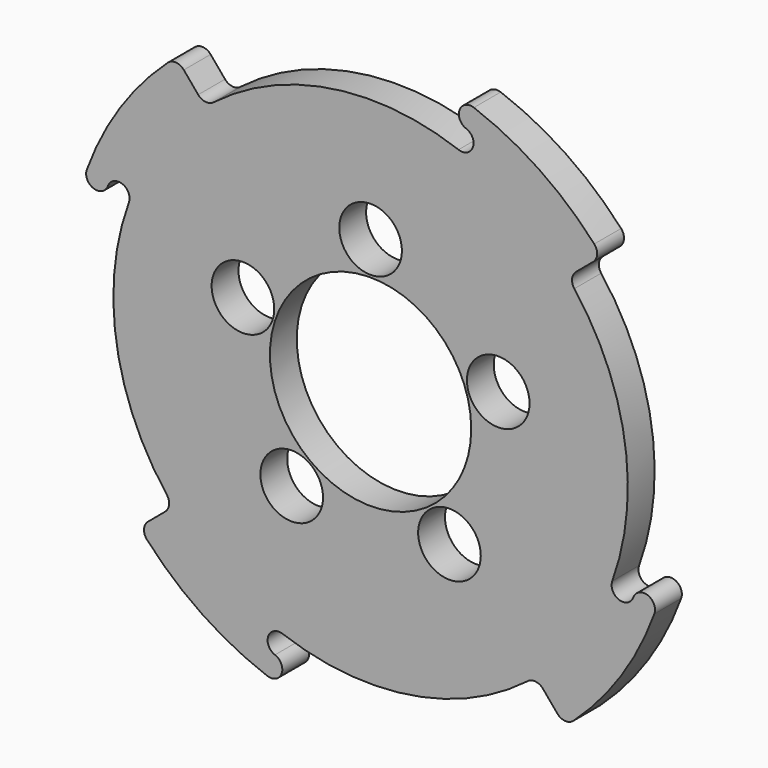
from build123d import *

# Parameters (mm, degrees)
F0_R     = 14
F0_R_2   = 45
F1_DEPTH = 15
F3_COUNT = 4
F4_R     = 14
F5_DEPTH = 15.001


# Not quite as in the source:
# - a feature names something its author has since deleted; it is built from what else it names


with BuildPart() as f1:
    # F0 (on Front) → F1 (new body)
    with BuildSketch(Plane.XZ):
        with BuildLine():
            ThreePointArc((-117.4615775982, 42.7525179157), (-111.0530137777, 45.740880303), (-108.0646513904, 39.3323164825))
            ThreePointArc((-108.0646513904, 39.3323164825), (-113.6444232454, -17.6052567496), (-91.0986302517, -70.1857504502))
            ThreePointArc((-91.0986302517, -70.1857504502), (-90.0886289945, -73.7767817278), (-91.8455022142, -77.0675270332))
            Line((-91.8455022142, -77.0675270332), (-99.5120922253, -83.500559884))
            ThreePointArc((-99.5120922253, -83.500559884), (-101.2865881138, -86.990889679), (-100.0019293376, -90.6896583342))
            ThreePointArc((-100.0019293376, -90.6896583342), (-75.2914558589, -112.0544362114), (-46.172719349, -126.8585038061))
            ThreePointArc((-46.172719349, -126.8585038061), (-39.7641555284, -123.8701414188), (-42.7525179157, -117.4615775982))
            ThreePointArc((-42.7525179157, -117.4615775982), (-45.740880303, -111.0530137777), (-39.3323164825, -108.0646513904))
            ThreePointArc((-39.3323164825, -108.0646513904), (17.6052567496, -113.6444232454), (70.1857504502, -91.0986302517))
            ThreePointArc((70.1857504502, -91.0986302517), (73.7767817278, -90.0886289945), (77.0675270332, -91.8455022142))
            Line((77.0675270332, -91.8455022142), (83.500559884, -99.5120922253))
            ThreePointArc((83.500559884, -99.5120922253), (86.990889679, -101.2865881138), (90.6896583342, -100.0019293376))
            ThreePointArc((90.6896583342, -100.0019293376), (112.0544362114, -75.2914558589), (126.8585038061, -46.172719349))
            ThreePointArc((126.8585038061, -46.172719349), (123.8701414188, -39.7641555284), (117.4615775982, -42.7525179157))
            ThreePointArc((117.4615775982, -42.7525179157), (111.0530137777, -45.740880303), (108.0646513904, -39.3323164825))
            ThreePointArc((108.0646513904, -39.3323164825), (113.6444232454, 17.6052567496), (91.0986302517, 70.1857504502))
            ThreePointArc((91.0986302517, 70.1857504502), (90.0886289945, 73.7767817278), (91.8455022142, 77.0675270332))
            Line((91.8455022142, 77.0675270332), (99.5120922253, 83.500559884))
            ThreePointArc((99.5120922253, 83.500559884), (101.2865881138, 86.990889679), (100.0019293376, 90.6896583342))
            ThreePointArc((100.0019293376, 90.6896583342), (75.2914558589, 112.0544362114), (46.172719349, 126.8585038061))
            ThreePointArc((46.172719349, 126.8585038061), (39.7641555284, 123.8701414188), (42.7525179157, 117.4615775982))
            ThreePointArc((42.7525179157, 117.4615775982), (45.740880303, 111.0530137777), (39.3323164825, 108.0646513904))
            ThreePointArc((39.3323164825, 108.0646513904), (-17.6052567496, 113.6444232454), (-70.1857504502, 91.0986302517))
            ThreePointArc((-70.1857504502, 91.0986302517), (-73.7767817278, 90.0886289945), (-77.0675270332, 91.8455022142))
            Line((-77.0675270332, 91.8455022142), (-83.500559884, 99.5120922253))
            ThreePointArc((-83.500559884, 99.5120922253), (-86.990889679, 101.2865881138), (-90.6896583342, 100.0019293376))
            ThreePointArc((-90.6896583342, 100.0019293376), (-112.0544362114, 75.2914558589), (-126.8585038061, 46.172719349))
            ThreePointArc((-126.8585038061, 46.172719349), (-123.8701414188, 39.7641555284), (-117.4615775982, 42.7525179157))
        make_face()
        with Locations((-35.2671151375, -48.5410196625)):
            Circle(F0_R, mode=Mode.SUBTRACT)
        with Locations((35.2671151375, -48.5410196625)):
            Circle(F0_R, mode=Mode.SUBTRACT)
        with Locations((-57.0633909777, 18.5410196625)):
            Circle(F0_R, mode=Mode.SUBTRACT)
        Circle(F0_R_2, mode=Mode.SUBTRACT)
        with Locations((57.0633909777, 18.5410196625)):
            Circle(F0_R, mode=Mode.SUBTRACT)
        with Locations((0, 60)):
            Circle(F0_R, mode=Mode.SUBTRACT)
    extrude(amount=F1_DEPTH)

    # F3: F1 ×4 about axis
    f3_axis = Axis((0, -15, 0), (0, -1, 0))


with BuildPart() as f1_1:
    add(f1.part)
    for i in range(1, F3_COUNT):
        add(f1.part.rotate(f3_axis, i * 360 / F3_COUNT))

    # F4 (on face) → F5 (cut, through all)
    with BuildSketch(Plane.XZ.offset(15)):
        with Locations((0, 60)):
            Circle(F4_R)
        with Locations((-57.0633909777, 18.5410196625)):
            Circle(F4_R)
        with Locations((-35.2671151375, -48.5410196625)):
            Circle(F4_R)
        with Locations((35.2671151375, -48.5410196625)):
            Circle(F4_R)
        with Locations((57.0633909777, 18.5410196625)):
            Circle(F4_R)
    extrude(amount=-F5_DEPTH, mode=Mode.SUBTRACT)


solid = f1_1.part
